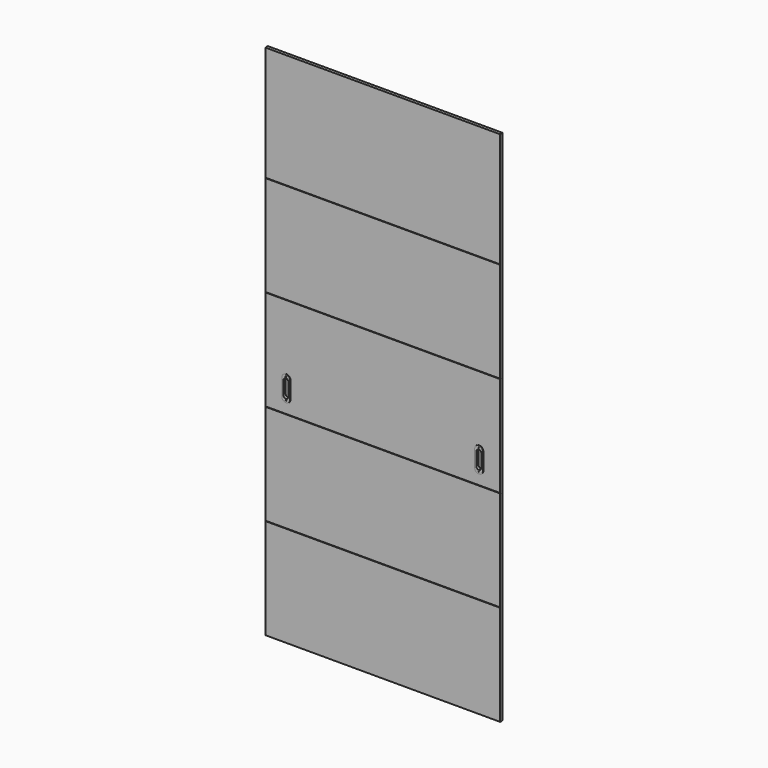
from build123d import *

# Parameters (mm, degrees)
F0_W      = 1120
F0_H      = 2467
F1_DEPTH  = 15
F3_DEPTH  = 1120.001
F5_DEPTH  = 13
F6_DEPTH  = 13
F7_START  = -11
F7_DEPTH  = 2
F4_R      = 1.75
F8_DEPTH  = 2
F9_DEPTH  = 2
F10_DEPTH = 2


with BuildPart() as f1:
    # F0 (on Front) → F1 (new body)
    with BuildSketch(Plane.XZ):
        with Locations((-101.7555719672, -4.3911735862)):
            Rectangle(F0_W, F0_H)
    extrude(amount=F1_DEPTH)

    # F2 (on face) → F3 (cut, through all)
    with BuildSketch(Plane(origin=(-661.7555719672, 0, 0), x_dir=(0, -1, 0), z_dir=(-1, 0, 0))):
        Polygon((15, -757.8911735862), (15, -756.8911735862), (14, -757.8911735862), (15, -758.8911735862), align=None)
        Polygon((15, 682.1088264138), (15, 683.1088264138), (14, 682.1088264138), (15, 681.1088264138), align=None)
        Polygon((14, -277.8911735862), (15, -278.8911735862), (15, -277.8911735862), (15, -276.8911735862), align=None)
        Polygon((14, 202.1088264138), (15, 201.1088264138), (15, 202.1088264138), (15, 203.1088264138), align=None)
    extrude(amount=-F3_DEPTH, mode=Mode.SUBTRACT)

    # F4 (on face) → F5 (cut)
    with BuildSketch(Plane.XZ.offset(15)):
        with BuildLine():
            Line((372.2444280328, -199.8911735862), (372.2444280328, -137.8911735862))
            ThreePointArc((372.2444280328, -137.8911735862), (358.2444280328, -123.8911735862), (344.2444280328, -137.8911735862))
            Line((344.2444280328, -137.8911735862), (344.2444280328, -199.8911735862))
            ThreePointArc((344.2444280328, -199.8911735862), (358.2444280328, -213.8911735862), (372.2444280328, -199.8911735862))
        make_face()
        with BuildLine():
            ThreePointArc((346.2444280328, -137.8911735862), (358.2444280328, -125.8911735862), (370.2444280328, -137.8911735862))
            Line((370.2444280328, -137.8911735862), (370.2444280328, -199.8911735862))
            ThreePointArc((370.2444280328, -199.8911735862), (358.2444280328, -211.8911735862), (346.2444280328, -199.8911735862))
            Line((346.2444280328, -199.8911735862), (346.2444280328, -137.8911735862))
        make_face(mode=Mode.SUBTRACT)
        with BuildLine():
            Line((-547.7555719672, -199.8911735862), (-547.7555719672, -137.8911735862))
            ThreePointArc((-547.7555719672, -137.8911735862), (-561.7555719672, -123.8911735862), (-575.7555719672, -137.8911735862))
            Line((-575.7555719672, -137.8911735862), (-575.7555719672, -199.8911735862))
            ThreePointArc((-575.7555719672, -199.8911735862), (-561.7555719672, -213.8911735862), (-547.7555719672, -199.8911735862))
        make_face()
        with BuildLine():
            ThreePointArc((-573.7555719672, -137.8911735862), (-561.7555719672, -125.8911735862), (-549.7555719672, -137.8911735862))
            Line((-549.7555719672, -137.8911735862), (-549.7555719672, -199.8911735862))
            ThreePointArc((-549.7555719672, -199.8911735862), (-561.7555719672, -211.8911735862), (-573.7555719672, -199.8911735862))
            Line((-573.7555719672, -199.8911735862), (-573.7555719672, -137.8911735862))
        make_face(mode=Mode.SUBTRACT)
        with BuildLine():
            Line((370.2444280328, -199.8911735862), (370.2444280328, -137.8911735862))
            ThreePointArc((370.2444280328, -137.8911735862), (358.2444280328, -125.8911735862), (346.2444280328, -137.8911735862))
            Line((346.2444280328, -137.8911735862), (346.2444280328, -199.8911735862))
            ThreePointArc((346.2444280328, -199.8911735862), (358.2444280328, -211.8911735862), (370.2444280328, -199.8911735862))
        make_face()
        with BuildLine():
            Line((-549.7555719672, -199.8911735862), (-549.7555719672, -137.8911735862))
            ThreePointArc((-549.7555719672, -137.8911735862), (-561.7555719672, -125.8911735862), (-573.7555719672, -137.8911735862))
            Line((-573.7555719672, -137.8911735862), (-573.7555719672, -199.8911735862))
            ThreePointArc((-573.7555719672, -199.8911735862), (-561.7555719672, -211.8911735862), (-549.7555719672, -199.8911735862))
        make_face()
    extrude(amount=-F5_DEPTH, mode=Mode.SUBTRACT)


with BuildPart() as f6:
    # F4 (on face) → F6 (new body)
    with BuildSketch(Plane.XZ.offset(15)):
        with BuildLine():
            Line((372.2444280328, -199.8911735862), (372.2444280328, -137.8911735862))
            ThreePointArc((372.2444280328, -137.8911735862), (358.2444280328, -123.8911735862), (344.2444280328, -137.8911735862))
            Line((344.2444280328, -137.8911735862), (344.2444280328, -199.8911735862))
            ThreePointArc((344.2444280328, -199.8911735862), (358.2444280328, -213.8911735862), (372.2444280328, -199.8911735862))
        make_face()
        with BuildLine():
            ThreePointArc((346.2444280328, -137.8911735862), (358.2444280328, -125.8911735862), (370.2444280328, -137.8911735862))
            Line((370.2444280328, -137.8911735862), (370.2444280328, -199.8911735862))
            ThreePointArc((370.2444280328, -199.8911735862), (358.2444280328, -211.8911735862), (346.2444280328, -199.8911735862))
            Line((346.2444280328, -199.8911735862), (346.2444280328, -137.8911735862))
        make_face(mode=Mode.SUBTRACT)
    extrude(amount=-F6_DEPTH)

    # F4 (on face) → F7 (join)
    with BuildSketch(Plane.XZ.offset(15).offset(F7_START)):
        with BuildLine():
            Line((370.2444280328, -199.8911735862), (370.2444280328, -137.8911735862))
            ThreePointArc((370.2444280328, -137.8911735862), (358.2444280328, -125.8911735862), (346.2444280328, -137.8911735862))
            Line((346.2444280328, -137.8911735862), (346.2444280328, -199.8911735862))
            ThreePointArc((346.2444280328, -199.8911735862), (358.2444280328, -211.8911735862), (370.2444280328, -199.8911735862))
        make_face()
    extrude(amount=-F7_DEPTH)

    # F4 (on face) → F8 (join)
    with BuildSketch(Plane.XZ.offset(15)):
        with BuildLine():
            Line((338.2444280328, -128.8911735862), (338.2444280328, -168.8911735862))
            Line((338.2444280328, -168.8911735862), (338.2444280328, -208.8911735862))
            ThreePointArc((338.2444280328, -208.8911735862), (344.1022924091, -223.03330921), (358.2444280328, -228.8911735862))
            ThreePointArc((358.2444280328, -228.8911735862), (372.3865636565, -223.03330921), (378.2444280328, -208.8911735862))
            Line((378.2444280328, -208.8911735862), (378.2444280328, -168.8911735862))
            Line((378.2444280328, -168.8911735862), (378.2444280328, -128.8911735862))
            ThreePointArc((378.2444280328, -128.8911735862), (372.3865636565, -114.7490379625), (358.2444280328, -108.8911735862))
            ThreePointArc((358.2444280328, -108.8911735862), (344.1022924091, -114.7490379625), (338.2444280328, -128.8911735862))
        make_face()
        with Locations((358.2444280328, -219.1505849063)):
            Circle(F4_R, mode=Mode.SUBTRACT)
        with BuildLine():
            ThreePointArc((344.2444280328, -137.8911735862), (358.2444280328, -123.8911735862), (372.2444280328, -137.8911735862))
            Line((372.2444280328, -137.8911735862), (372.2444280328, -199.8911735862))
            ThreePointArc((372.2444280328, -199.8911735862), (358.2444280328, -213.8911735862), (344.2444280328, -199.8911735862))
            Line((344.2444280328, -199.8911735862), (344.2444280328, -137.8911735862))
        make_face(mode=Mode.SUBTRACT)
        with Locations((358.2444280328, -118.6317622662)):
            Circle(F4_R, mode=Mode.SUBTRACT)
        with BuildLine():
            Line((372.2444280328, -199.8911735862), (372.2444280328, -137.8911735862))
            ThreePointArc((372.2444280328, -137.8911735862), (358.2444280328, -123.8911735862), (344.2444280328, -137.8911735862))
            Line((344.2444280328, -137.8911735862), (344.2444280328, -199.8911735862))
            ThreePointArc((344.2444280328, -199.8911735862), (358.2444280328, -213.8911735862), (372.2444280328, -199.8911735862))
        make_face()
        with BuildLine():
            ThreePointArc((346.2444280328, -137.8911735862), (358.2444280328, -125.8911735862), (370.2444280328, -137.8911735862))
            Line((370.2444280328, -137.8911735862), (370.2444280328, -199.8911735862))
            ThreePointArc((370.2444280328, -199.8911735862), (358.2444280328, -211.8911735862), (346.2444280328, -199.8911735862))
            Line((346.2444280328, -199.8911735862), (346.2444280328, -137.8911735862))
        make_face(mode=Mode.SUBTRACT)
    extrude(amount=F8_DEPTH)


with BuildPart() as f6b:
    # F4 (on face) → F6, piece 2 (new body)
    with BuildSketch(Plane.XZ.offset(15)):
        with BuildLine():
            Line((-547.7555719672, -199.8911735862), (-547.7555719672, -137.8911735862))
            ThreePointArc((-547.7555719672, -137.8911735862), (-561.7555719672, -123.8911735862), (-575.7555719672, -137.8911735862))
            Line((-575.7555719672, -137.8911735862), (-575.7555719672, -199.8911735862))
            ThreePointArc((-575.7555719672, -199.8911735862), (-561.7555719672, -213.8911735862), (-547.7555719672, -199.8911735862))
        make_face()
        with BuildLine():
            ThreePointArc((-573.7555719672, -137.8911735862), (-561.7555719672, -125.8911735862), (-549.7555719672, -137.8911735862))
            Line((-549.7555719672, -137.8911735862), (-549.7555719672, -199.8911735862))
            ThreePointArc((-549.7555719672, -199.8911735862), (-561.7555719672, -211.8911735862), (-573.7555719672, -199.8911735862))
            Line((-573.7555719672, -199.8911735862), (-573.7555719672, -137.8911735862))
        make_face(mode=Mode.SUBTRACT)
    extrude(amount=-F6_DEPTH)

    # F9 (add): a face of the model
    f9_faces = [f1.part.faces().sort_by_distance(p)[0] for p in [
        (-561.7555719672, -2, -168.8911735862),
    ]]
    extrude(f9_faces, amount=F9_DEPTH)

    # F4 (on face) → F10 (join)
    with BuildSketch(Plane.XZ.offset(15)):
        with BuildLine():
            Line((-581.7555719672, -128.8911735862), (-581.7555719672, -168.8911735862))
            Line((-581.7555719672, -168.8911735862), (-581.7555719672, -208.8911735862))
            ThreePointArc((-581.7555719672, -208.8911735862), (-575.8977075909, -223.03330921), (-561.7555719672, -228.8911735862))
            ThreePointArc((-561.7555719672, -228.8911735862), (-547.6134363435, -223.03330921), (-541.7555719672, -208.8911735862))
            Line((-541.7555719672, -208.8911735862), (-541.7555719672, -168.8911735862))
            Line((-541.7555719672, -168.8911735862), (-541.7555719672, -128.8911735862))
            ThreePointArc((-541.7555719672, -128.8911735862), (-547.6134363435, -114.7490379625), (-561.7555719672, -108.8911735862))
            ThreePointArc((-561.7555719672, -108.8911735862), (-575.8977075909, -114.7490379625), (-581.7555719672, -128.8911735862))
        make_face()
        with Locations((-561.7555719672, -219.1505849063)):
            Circle(F4_R, mode=Mode.SUBTRACT)
        with BuildLine():
            ThreePointArc((-575.7555719672, -137.8911735862), (-561.7555719672, -123.8911735862), (-547.7555719672, -137.8911735862))
            Line((-547.7555719672, -137.8911735862), (-547.7555719672, -199.8911735862))
            ThreePointArc((-547.7555719672, -199.8911735862), (-561.7555719672, -213.8911735862), (-575.7555719672, -199.8911735862))
            Line((-575.7555719672, -199.8911735862), (-575.7555719672, -137.8911735862))
        make_face(mode=Mode.SUBTRACT)
        with Locations((-561.7555719672, -118.6317622662)):
            Circle(F4_R, mode=Mode.SUBTRACT)
        with BuildLine():
            Line((-547.7555719672, -199.8911735862), (-547.7555719672, -137.8911735862))
            ThreePointArc((-547.7555719672, -137.8911735862), (-561.7555719672, -123.8911735862), (-575.7555719672, -137.8911735862))
            Line((-575.7555719672, -137.8911735862), (-575.7555719672, -199.8911735862))
            ThreePointArc((-575.7555719672, -199.8911735862), (-561.7555719672, -213.8911735862), (-547.7555719672, -199.8911735862))
        make_face()
        with BuildLine():
            ThreePointArc((-573.7555719672, -137.8911735862), (-561.7555719672, -125.8911735862), (-549.7555719672, -137.8911735862))
            Line((-549.7555719672, -137.8911735862), (-549.7555719672, -199.8911735862))
            ThreePointArc((-549.7555719672, -199.8911735862), (-561.7555719672, -211.8911735862), (-573.7555719672, -199.8911735862))
            Line((-573.7555719672, -199.8911735862), (-573.7555719672, -137.8911735862))
        make_face(mode=Mode.SUBTRACT)
    extrude(amount=F10_DEPTH)


solid = Compound([f1.part, f6.part, f6b.part])
